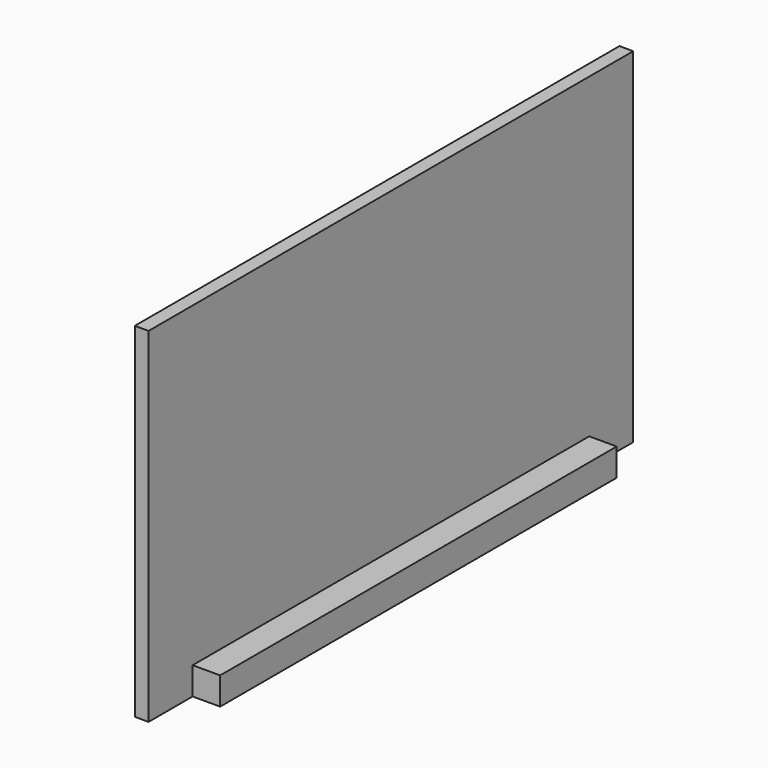
from build123d import *

# Parameters (mm, degrees)
F0_W     = 15
F0_H     = 20
F1_DEPTH = 15
F2_W     = 220
F2_H     = 125
F2_W_2   = 15
F2_H_2   = 55
F3_DEPTH = 5
F4_W     = 180
F4_H     = 10
F5_DEPTH = 10


with BuildPart() as f1:
    # F0 (on Front) → F1 (new body)
    with BuildSketch(Plane.XZ):
        with Locations((12.5, 17.5)):
            Rectangle(F0_W, F0_H)
        with Locations((12.5, -17.5)):
            Rectangle(F0_W, F0_H)
        Polygon((5, 7.5), (-20, 7.5), (-20, -7.5), (5, -7.5), (20, -7.5), (20, 7.5), align=None)
    extrude(amount=F1_DEPTH)

    # F2 (on face) → F3 (join)
    with BuildSketch(Plane.YZ.offset(20)):
        with Locations((-7.5, 0)):
            Rectangle(F2_W, F2_H)
        with Locations((-7.5, 0)):
            Rectangle(F2_W_2, F2_H_2, mode=Mode.SUBTRACT)
        with Locations((-7.5, 0)):
            Rectangle(F2_W_2, F2_H_2)
    extrude(amount=F3_DEPTH)

    # F4 (on face) → F5 (join)
    with BuildSketch(Plane.YZ.offset(25)):
        with Locations((-7.5, -57.5)):
            Rectangle(F4_W, F4_H)
    extrude(amount=F5_DEPTH)


solid = f1.part
